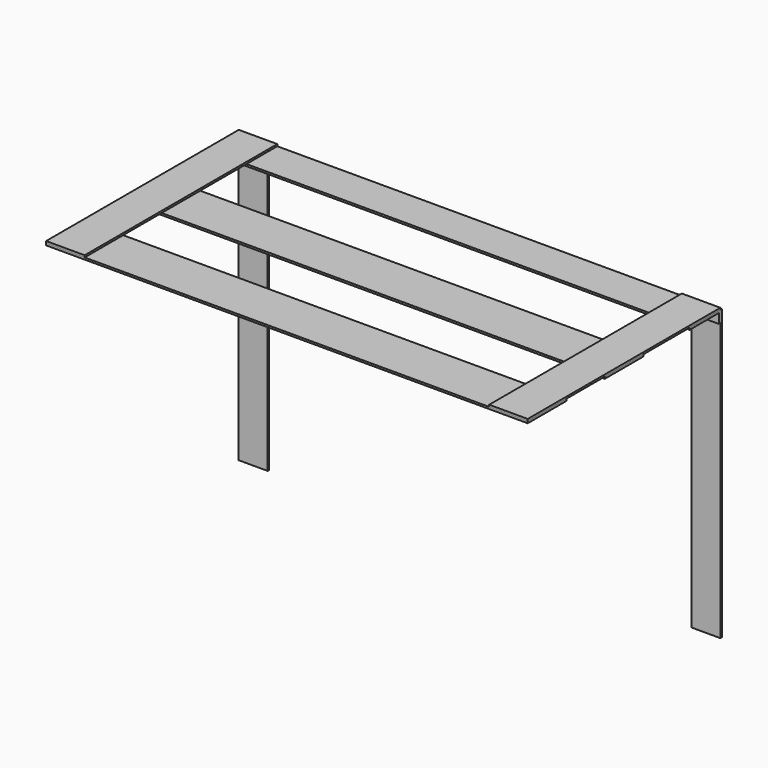
from build123d import *

# Parameters (mm, degrees)
F0_W      = 500
F0_H      = 40
F1_DEPTH  = 2
F2_W      = 40
F2_H      = 250
F3_DEPTH  = 2
F4_W      = 500
F4_H      = 50
F5_DEPTH  = 2
F7_W      = 500
F7_H      = 2
F8_DEPTH  = 10
F9_W      = 30
F9_H      = 300
F10_DEPTH = 2


# Not quite as in the source:
# - a feature names something its author has since deleted; it is built from what else it names


with BuildPart() as f1:
    # F0 (on Top) → F1 (new body)
    with BuildSketch(Plane.XY):
        with Locations((-1.1249929667, 207.531722784)):
            Rectangle(F0_W, F0_H)
    extrude(amount=-F1_DEPTH)

    # F7 (on face) → F8 (join)
    with BuildSketch(Plane(origin=(0, 0, -2), x_dir=(1, 0, 0), z_dir=(0, 0, -1))):
        with Locations((-1.1249929667, -226.531722784)):
            Rectangle(F7_W, F7_H)
    extrude(amount=F8_DEPTH)

    # F9 (on face) → F10 (join)
    with BuildSketch(Plane(origin=(0, 227.531722784, 0), x_dir=(-1, 0, 0), z_dir=(0, 1, 0))):
        with Locations((-233.8750070333, -150)):
            Rectangle(F9_W, F9_H)
        with Locations((236.1249929667, -150)):
            Rectangle(F9_W, F9_H)
    extrude(amount=F10_DEPTH)


with BuildPart() as f3:
    # F2 (on Top) → F3 (new body)
    with BuildSketch(Plane.XY):
        with Locations((-231.1249929667, 102.531722784)):
            Rectangle(F2_W, F2_H)
    extrude(amount=F3_DEPTH)


with BuildPart() as f3b:
    # F2 (on Top) → F3, piece 2 (new body)
    with BuildSketch(Plane.XY):
        with Locations((228.8750070333, 102.531722784)):
            Rectangle(F2_W, F2_H)
    extrude(amount=F3_DEPTH)


with BuildPart() as f5:
    # F4 (on Top) → F5 (new body)
    with BuildSketch(Plane.XY):
        with Locations((-1.1249929667, 2.531722784)):
            Rectangle(F4_W, F4_H)
    extrude(amount=-F5_DEPTH)


with BuildPart() as f5b:
    # F4 (on Top) → F5, piece 2 (new body)
    with BuildSketch(Plane.XY):
        with Locations((-1.1249929667, 102.531722784)):
            Rectangle(F4_W, F4_H)
    extrude(amount=-F5_DEPTH)


solid = Compound([f1.part, f3.part, f3b.part, f5.part, f5b.part])
